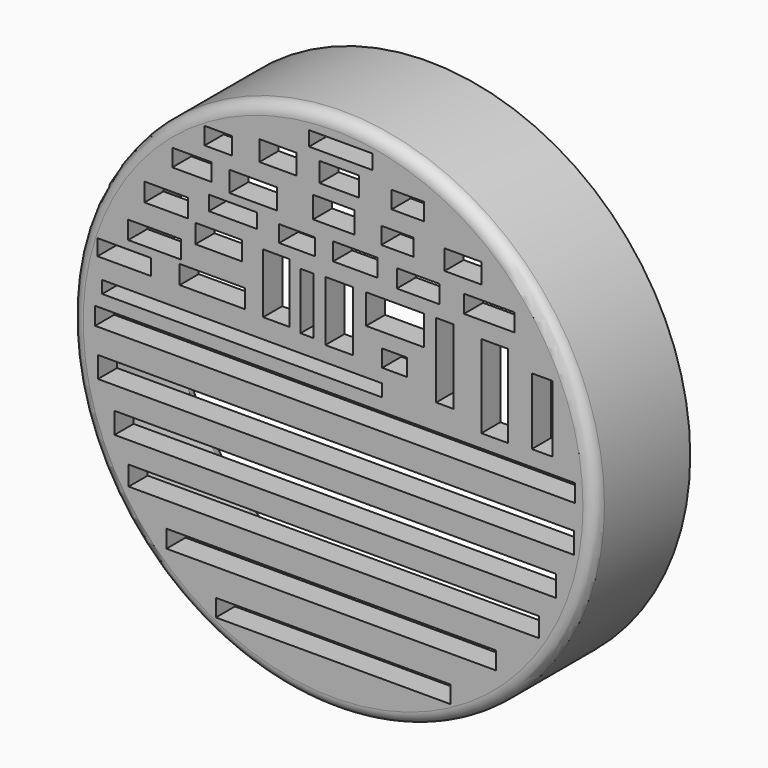
from build123d import *

# Parameters (mm, degrees)
F0_R     = 55.8162031388
F0_R_2   = 53.34
F1_DEPTH = 25.4
F2_DEPTH = 5.08
F3_W     = 13.5487690568
F3_H     = 3.1119100749
F3_W_2   = 8.3945244551
F3_H_2   = 4.1670650244
F3_W_3   = 7.9046934843
F3_H_3   = 4.2887181044
F3_W_4   = 5.7976543903
F3_H_4   = 3.6839321256
F3_W_5   = 8.4092468023
F3_H_5   = 3.7000700831
F3_W_6   = 10.0910961628
F3_H_6   = 4.372805357
F3_W_7   = 8.8297128677
F3_H_7   = 4.6250857413
F3_W_8   = 6.8733096123
F3_H_8   = 3.6097243428
F3_W_9   = 6.8847164512
F3_H_9   = 3.6839284003
F3_W_10  = 7.9117268324
F3_H_10  = 4.2525529861
F3_W_11  = 10.2453604341
F3_H_11  = 3.1119063497
F3_W_12  = 9.3357227743
F3_H_12  = 3.9257928729
F3_W_13  = 9.9581070244
F3_H_13  = 4.0215402842
F3_W_14  = 13.9796473086
F3_H_14  = 3.9736665785
F3_W_15  = 11.2507455051
F3_H_15  = 3.8300380111
F3_W_16  = 11.3943703473
F3_H_16  = 3.3991634846
F3_W_17  = 7.6600834727
F3_H_17  = 3.5427883267
F3_W_18  = 9.4169080257
F3_H_18  = 3.7821643054
F3_W_19  = 9.1442242265
F3_H_19  = 3.8300417364
F3_W_20  = 10.7719898224
F3_W_21  = 5.6493058801
F3_H_20  = 12.7348862588
F3_W_22  = 2.7767792344
F3_H_21  = 12.112505734
F3_W_23  = 5.8886855841
F3_H_22  = 12.7827599645
F3_W_24  = 12.351885438
F3_H_23  = 6.3195675611
F3_W_25  = 5.2663087845
F3_H_24  = 3.6385394633
F3_W_26  = 3.6878287792
F3_H_25  = 15.8802717924
F3_W_27  = 5.7199150324
F3_H_26  = 17.6865570247
F3_W_28  = 4.3651908636
F3_H_27  = 14.2245069146
F3_W_29  = 59.7025379539
F3_H_28  = 2.6341676712
F3_W_30  = 102.2809818387
F3_H_29  = 3.7544369698
F3_W_31  = 101.4531031251
F3_H_30  = 4.5157186687
F3_W_32  = 50.049200654
F3_H_31  = 3.6878362298
F3_W_33  = 70.2946484089
F3_H_32  = 3.7630945444
F3_W_34  = 87.4543711543
F3_H_33  = 4.1394084692
F3_W_35  = 94.1526964307
F3_H_34  = 4.5157149434
F4_DEPTH = 25.4


# Not quite as in the source:
# - a fillet or chamfer that OpenCascade refuses, or shapes differently, is made with other operations: its cross-section is extruded or revolved along the edge and cut away or added


with BuildPart() as f1:
    # F0 (on Front) → F1 (new body)
    with BuildSketch(Plane.XZ):
        Circle(F0_R)
        Circle(F0_R_2, mode=Mode.SUBTRACT)
    extrude(amount=-F1_DEPTH)

    # F0 (on Front) → F2 (join)
    with BuildSketch(Plane.XZ):
        Circle(F0_R_2)
    extrude(amount=-F2_DEPTH)

    # F3 (on face) → F4 (cut)
    with BuildSketch(Plane.XZ):
        with Locations((1.637134701, 50.0085186213)):
            Rectangle(F3_W, F3_H)
        with Locations((1.3199597597, 44.4235429168)):
            Rectangle(F3_W_2, F3_H_2)
        with Locations((-11.756375432, 44.2828312516)):
            Rectangle(F3_W_3, F3_H_3)
        with Locations((-24.4977399707, 43.2760901749)):
            Rectangle(F3_W_4, F3_H_4)
        with Locations((-30.0885364413, 36.9247384369)):
            Rectangle(F3_W_5, F3_H_5)
        with Locations((-17.0542001724, 36.4201851189)):
            Rectangle(F3_W_6, F3_H_6)
        with Locations((0.1427084208, 37.387246266)):
            Rectangle(F3_W_7, F3_H_7)
        with Locations((13.7023478746, 36.8178598583)):
            Rectangle(F3_W_8, F3_H_8)
        with Locations((15.9046910703, 44.2423652858)):
            Rectangle(F3_W_9, F3_H_9)
        with Locations((27.7209356427, 36.6447903216)):
            Rectangle(F3_W_10, F3_H_10)
        with Locations((-21.367046982, 30.954066664)):
            Rectangle(F3_W_11, F3_H_11)
        with Locations((-35.5621371418, 28.5363532603)):
            Rectangle(F3_W_12, F3_H_12)
        with Locations((-24.3832040578, 24.2754332721)):
            Rectangle(F3_W_13, F3_H_13)
        with Locations((-25.7237199694, 15.490276739)):
            Rectangle(F3_W_14, F3_H_14)
        with Locations((-38.0516629666, 20.3017666936)):
            Rectangle(F3_W_15, F3_H_15)
        with Locations((-44.5387940854, 14.9157717824)):
            Rectangle(F3_W_16, F3_H_16)
        with Locations((-7.6746530831, 30.0683714449)):
            Rectangle(F3_W_17, F3_H_17)
        with Locations((4.7084540129, 30.4753128439)):
            Rectangle(F3_W_18, F3_H_18)
        with Locations((18.1541852653, 29.8289936036)):
            Rectangle(F3_W_19, F3_H_19)
        with Locations((33.2828462124, 29.7093037516)):
            Rectangle(F3_W_20, F3_H_18)
        with Locations((-12.0791979134, 19.6315106004)):
            Rectangle(F3_W_21, F3_H_20)
        with Locations((-5.5681280792, 18.8894383609)):
            Rectangle(F3_W_22, F3_H_21)
        with Locations((1.3020038605, 18.7458135188)):
            Rectangle(F3_W_23, F3_H_22)
        with Locations((13.1990686059, 21.9295322895)):
            Rectangle(F3_W_24, F3_H_23)
        with Locations((13.1033211946, 13.8385724276)):
            Rectangle(F3_W_25, F3_H_24)
        with Locations((23.8093435764, 17.1886943281)):
            Rectangle(F3_W_26, F3_H_25)
        with Locations((34.458912909, 15.457669273)):
            Rectangle(F3_W_27, F3_H_26)
        with Locations((44.544018805, 14.2534784973)):
            Rectangle(F3_W_28, F3_H_27)
        with Locations((-19.3811021745, 7.7809505165)):
            Rectangle(F3_W_29, F3_H_28)
        with Locations((0.4028789699, 1.8772184849)):
            Rectangle(F3_W_30, F3_H_29)
        with Locations((0.5910359323, -7.5348559767)):
            Rectangle(F3_W_31, F3_H_30)
        with Locations((0.026576221, -44.526103884)):
            Rectangle(F3_W_32, F3_H_31)
        with Locations((-0.3873705864, -35.0054651499)):
            Rectangle(F3_W_33, F3_H_32)
        with Locations((0.1394636929, -25.7858783007)):
            Rectangle(F3_W_34, F3_H_33)
        with Locations((0.4781447351, -16.8673358858)):
            Rectangle(F3_W_35, F3_H_34)
    extrude(amount=-F4_DEPTH, mode=Mode.SUBTRACT)

    # F5: fillet of radius 2.54 on 2 edges, made by hand

    # F5_s1 → F5_t2 (revolve, cut)
    with BuildSketch(Plane.XY):
        with BuildLine():
            ThreePointArc((55.8162031388, 2.54), (55.072254363, 0.7439487758), (53.2762031388, 0))
            Line((53.2762031388, 0), (55.8162031388, 0))
            Line((55.8162031388, 0), (55.8162031388, 2.54))
        make_face()
    revolve(axis=Axis((0, 0, 0), (0, -1, 0)), mode=Mode.SUBTRACT)

    # F5_s3 → F5_t4 (revolve, cut)
    with BuildSketch(Plane.XY):
        with BuildLine():
            ThreePointArc((55.88, 25.4), (54.0839487758, 24.6560512242), (53.34, 22.86))
            Line((53.34, 22.86), (53.34, 25.4))
            Line((53.34, 25.4), (55.88, 25.4))
        make_face()
    revolve(axis=Axis((0, 25.4, 0), (0, -1, 0)), mode=Mode.SUBTRACT)


solid = f1.part
